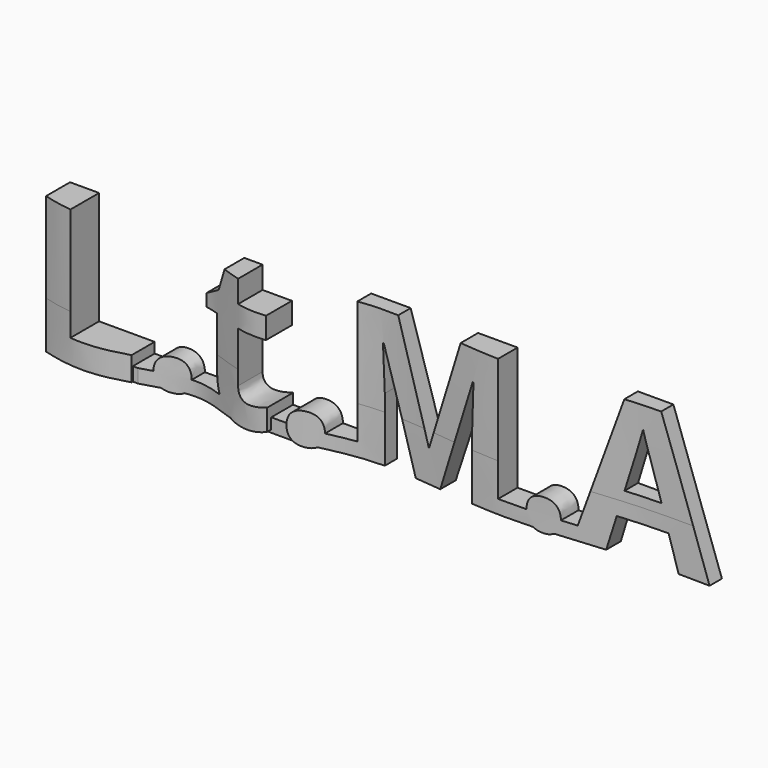
from build123d import *

# Parameters (mm, degrees)
F0_TEXT_SIZE  = 14.3010468901
F1_DEPTH      = 3.175
F2_W          = 7.3181355322
F2_H          = 1.016
F2_W_2        = 6.466400286
F2_W_3        = 5.720087004
F3_DEPTH      = 2.032
F5_DEPTH      = 3.7011465124
F5_DEPTH_BACK = 6.7406179174


# Not quite as in the source:
# - a feature of the source that left no trace in its solid (it failed there, or was rolled back) is left out
# - Text() gives the source's letters only with a copy of the font that has no kerning and outlines rounded to 1/6400 em; it was checked with that copy


with BuildPart() as f1:
    # F0 (on Front) → F1 (new body)
    with BuildSketch(Plane.XZ):
        with Locations((-25.9343488131, -3.512445172)):
            Text('L.t.M.A', F0_TEXT_SIZE, font='Open Sans', font_style=FontStyle.BOLD, text_align=(TextAlign.LEFT, TextAlign.BOTTOM))
    extrude(amount=F1_DEPTH)

    # F2 (on Front) → F3 (join)
    with BuildSketch(Plane.XZ):
        with Locations((-14.6845535023, -3.004445172)):
            Rectangle(F2_W, F2_H)
        with Locations((-5.4389838114, -3.004445172)):
            Rectangle(F2_W_2, F2_H)
        with Locations((11.5677462417, -3.004445172)):
            Rectangle(F2_W_3, F2_H)
    extrude(amount=F3_DEPTH)

    # F4 (on Top) → F5 (cut, two sides)
    with BuildSketch(Plane.XY) as f5_sk:
        with BuildLine():
            add(Edge.make_bspline(
                [(-27.563014999, -1.2215980096), (-25.3246583233, -2.066876799), (-20.8797477331, -3.7454245852), (-14.1215413553, -0.0848148941), (-9.4172368106, -3.5367767282), (-1.4300596189, -0.2227681722), (8.1402212526, -2.450647443), (18.1384919885, -0.9848674855), (22.9724546962, -1.1233417148), (25.164924562, -1.1861474486)],
                knots=[0, 0, 0, 0, 0.1372966282, 0.2726425344, 0.3879939605, 0.5338756399, 0.6979654416, 0.8630105965, 1, 1, 1, 1], degree=3))
            Line((-27.563014999, -1.2215980096), (-27.563014999, -4.9605965614))
            Line((-27.563014999, -4.9605965614), (25.3221932799, -4.9605965614))
            Line((25.3221932799, -4.9605965614), (25.164924562, -1.1861474486))
        make_face()
    extrude(amount=-F5_DEPTH, mode=Mode.SUBTRACT)
    extrude(f5_sk.sketch, amount=F5_DEPTH_BACK, mode=Mode.SUBTRACT)


solid = f1.part
